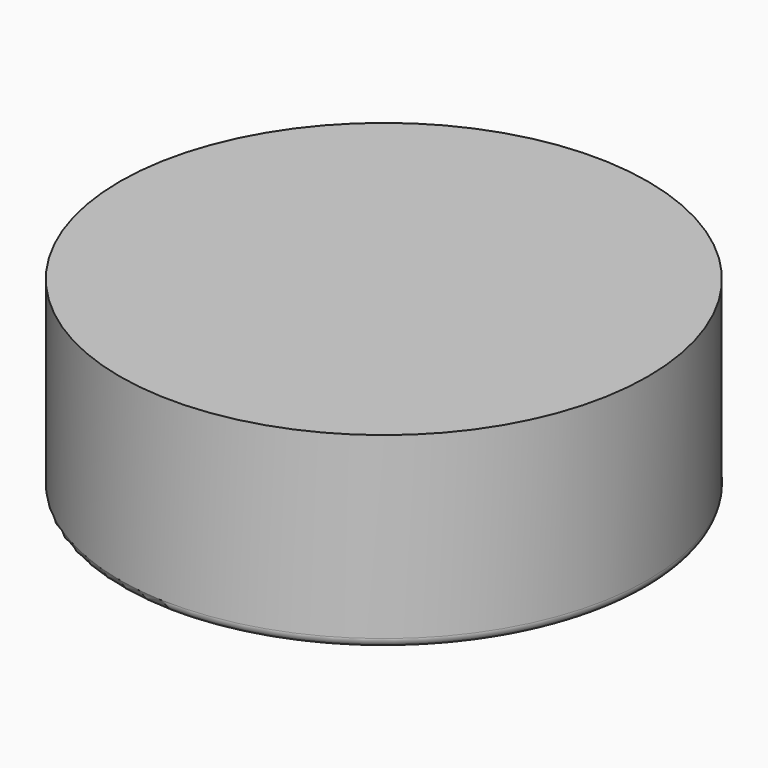
from build123d import *

# Parameters (mm, degrees)
F2_R = 0.99999
F3_R = 0.5


# Not quite as in the source:
# - a fillet or chamfer is up to 0.001 mm smaller than in the source, because OpenCascade refuses the exact size


with BuildPart() as f1:
    # F0 (on Front) → F1 (revolve)
    with BuildSketch(Plane.XZ):
        Polygon((19.1826918498, 16.5195801589), (-8.8173081502, 16.5195801589), (-8.8173081502, -3.4804198411), (-6.8173081502, -3.4804198411), (-6.8173081502, 14.5195801589), (19.1826918498, 14.5195801589), align=None)
    revolve(axis=Axis((19.1826918498, 0, 15.5195801589), (0, 0, -1)))

    # F2 (radius 1 in the source; OpenCascade refuses exactly that, so slightly less here)
    f2_edges = [f1.edges().sort_by_distance(p)[0] for p in [
        (47.182692, 0, -3.48042),
        (45.182692, 0, -3.48042),
    ]]
    fillet(f2_edges, radius=F2_R)

    # F3
    f3_edges = [f1.edges().sort_by_distance(p)[0] for p in [
        (45.182692, 0, 14.51958),
    ]]
    fillet(f3_edges, radius=F3_R)


solid = f1.part
